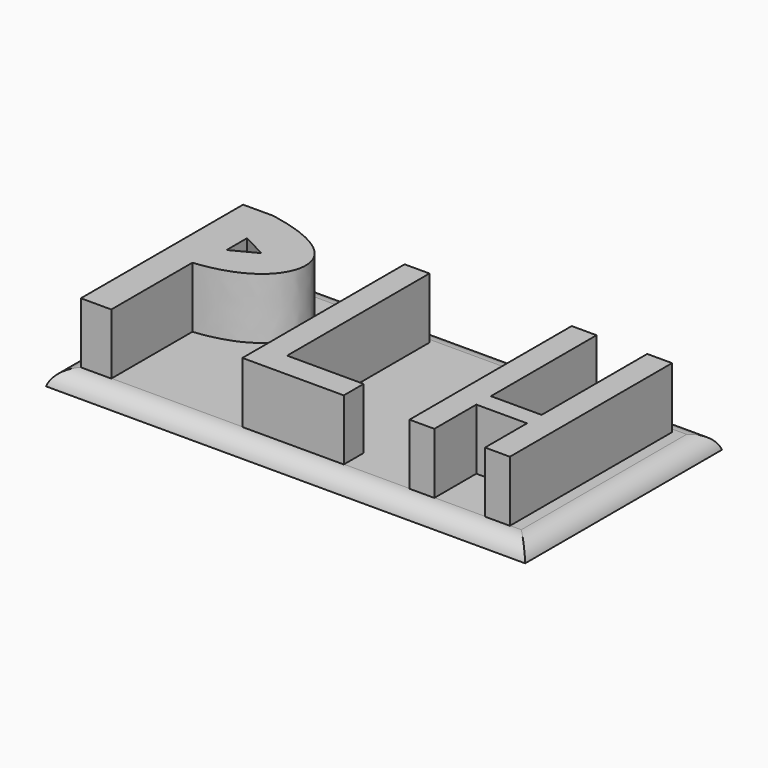
from build123d import *

# Parameters (mm, degrees)
F1_DEPTH    = 15.24
F2_DEPTH    = 15.24
F0_W        = 6.223
F0_H        = 44.577
F0_H_2      = 6.223
F0_W_2      = 19.177
F4_DEPTH    = 3.81
F5_T1_DEPTH = 144.6338988167
F5_T3_DEPTH = 86.212517401


# Not quite as in the source:
# - a fillet or chamfer that OpenCascade refuses, or shapes differently, is made with other operations: its cross-section is extruded or revolved along the edge and cut away or added


with BuildPart() as f1:
    # F0 (on Top) → F1 (new body)
    with BuildSketch(Plane.XY):
        with BuildLine():
            add(Edge.make_bspline(
                [(-58.2525283742, 33.0758240239), (-45.5206043265, 30.688588265), (-34.6846427624, 21.2199367045), (-45.8849792124, 8.8536855352), (-58.2525283742, 7.6758240239)],
                knots=[0, 0, 0, 0, 0.4990909505, 1, 1, 1, 1], degree=3))
            Line((-58.2525283742, 33.0758240239), (-65.8725283742, 33.0758240239))
            Line((-65.8725283742, 33.0758240239), (-65.8725283742, -17.7241759761))
            Line((-65.8725283742, -17.7241759761), (-58.2525283742, -17.7241759761))
            Line((-58.2525283742, -17.7241759761), (-58.2525283742, 7.6758240239))
        make_face()
        Polygon((-56.3824130938, 16.0494490157), (-56.3824130938, 22.4692318326), (-50.2417553016, 19.2593404241), align=None, mode=Mode.SUBTRACT)
    extrude(amount=F1_DEPTH)

    # F0 (on Top) → F2 (join)
    with BuildSketch(Plane.XY):
        with BuildLine():
            add(Edge.make_bspline(
                [(-58.2525283742, 33.0758240239), (-45.5206043265, 30.688588265), (-34.6846427624, 21.2199367045), (-45.8849792124, 8.8536855352), (-58.2525283742, 7.6758240239)],
                knots=[0, 0, 0, 0, 0.4990909505, 1, 1, 1, 1], degree=3))
            Line((-58.2525283742, 33.0758240239), (-65.8725283742, 33.0758240239))
            Line((-65.8725283742, 33.0758240239), (-65.8725283742, -17.7241759761))
            Line((-65.8725283742, -17.7241759761), (-58.2525283742, -17.7241759761))
            Line((-58.2525283742, -17.7241759761), (-58.2525283742, 7.6758240239))
        make_face()
        Polygon((-56.3824130938, 16.0494490157), (-56.3824130938, 22.4692318326), (-50.2417553016, 19.2593404241), align=None, mode=Mode.SUBTRACT)
    extrude(amount=F2_DEPTH)


with BuildPart() as f2:
    # F0 (on Top) → F2, piece 2 (new body)
    with BuildSketch(Plane.XY):
        with Locations((-22.2885, 10.7873240239)):
            Rectangle(F0_W, F0_H)
        with Locations((-22.2885, -14.6126759761)):
            Rectangle(F0_W, F0_H_2)
        with Locations((-9.5885, -14.6126759761)):
            Rectangle(F0_W_2, F0_H_2)
    extrude(amount=F2_DEPTH)


with BuildPart() as f2b:
    # F0 (on Top) → F2, piece 3 (new body)
    with BuildSketch(Plane.XY):
        Polygon((22.6911320935, 33.0758240239), (16.4681320935, 33.0758240239), (16.4681320935, -17.7241759761), (22.6911320935, -17.7241759761), (22.6911320935, -4.572), (35.3911320935, -4.572), (35.3911320935, -17.7241759761), (41.6141320935, -17.7241759761), (41.6141320935, 33.0758240239), (35.3911320935, 33.0758240239), (35.3911320935, 0), (22.6911320935, 0), align=None)
    extrude(amount=F2_DEPTH)


with BuildPart() as f4:
    # F3 (on Top) → F4 (new body)
    with BuildSketch(Plane.XY):
        Polygon((49.3206983823, -17.523912622), (49.3206983823, 32.3124918177), (49.3206983823, 39.0570126474), (-70.719756186, 39.0570126474), (-70.719756186, -22.5620605052), (49.3206983823, -22.5620605052), align=None)
    extrude(amount=-F4_DEPTH)

    # F5: fillet of radius 5.08 on 4 edges, made by hand

    # F5_s2 → F5_t1 (cut)
    with BuildSketch(Plane.YZ.offset(-83.0164783102)):
        with BuildLine():
            ThreePointArc((-17.6433716555, 0), (-20.7542236288, -1.0639073716), (-22.5620605052, -3.81))
            Line((-22.5620605052, -3.81), (-22.5620605052, 0))
            Line((-22.5620605052, 0), (-17.6433716555, 0))
        make_face()
        with BuildLine():
            ThreePointArc((34.1383237977, 0), (37.249175771, -1.0639073716), (39.0570126474, -3.81))
            Line((39.0570126474, -3.81), (39.0570126474, 0))
            Line((39.0570126474, 0), (34.1383237977, 0))
        make_face()
    extrude(amount=F5_T1_DEPTH, mode=Mode.SUBTRACT)

    # F5_s4 → F5_t3 (cut)
    with BuildSketch(Plane.XZ.offset(-51.3537347716)):
        with BuildLine():
            ThreePointArc((-65.8010673363, 0), (-68.9119193097, -1.0639073716), (-70.719756186, -3.81))
            Line((-70.719756186, -3.81), (-70.719756186, 0))
            Line((-70.719756186, 0), (-65.8010673363, 0))
        make_face()
        with BuildLine():
            ThreePointArc((49.3206983823, -3.81), (47.512861506, -1.0639073716), (44.4020095326, 0))
            Line((44.4020095326, 0), (49.3206983823, 0))
            Line((49.3206983823, 0), (49.3206983823, -3.81))
        make_face()
    extrude(amount=F5_T3_DEPTH, mode=Mode.SUBTRACT)


solid = Compound([f1.part, f2.part, f2b.part, f4.part])
